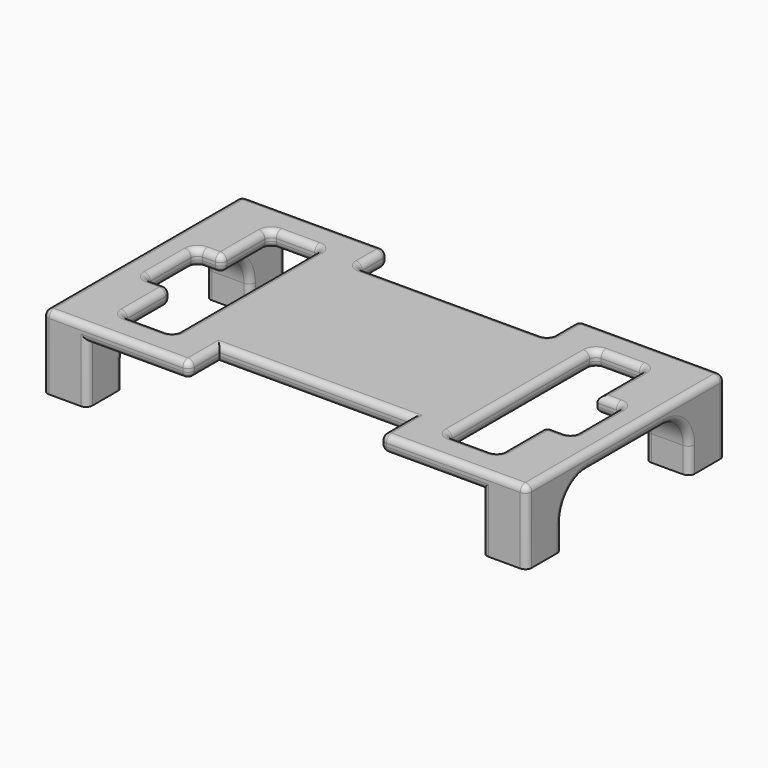
from build123d import *

# Parameters (mm, degrees)
F0_W     = 7
F0_H     = 7
F0_R     = 1.5
F0_R_2   = 1.325
F1_DEPTH = 9
F2_START = 9
F2_DEPTH = 2.5
F4_R     = 5
F5_W     = 4
F5_H     = 10
F5_W_2   = 30
F5_H_2   = 6
F6_DEPTH = 10
F7_F1_R  = 1
F7_F2_R  = 1
F7_F3_R  = 1
F7_F4_R  = 1
F7_F5_R  = 1
F7_F6_R  = 1
F7_F7_R  = 1
F7_F8_R  = 1
F7_F9_R  = 1
F7_F10_R = 1
F7_F11_R = 1
F7_F12_R = 1
F7_F13_R = 1
F7_F14_R = 1
F7_F15_R = 1
F7_F16_R = 1
F7_F17_R = 1
F7_F18_R = 1
F7_F19_R = 1
F7_F20_R = 1
F7_F21_R = 1
F7_F22_R = 1
F7_F23_R = 1
F7_F24_R = 1
F7_F25_R = 1
F7_F26_R = 1
F7_F27_R = 1
F7_F28_R = 1
F7_F29_R = 1
F7_F30_R = 1
F7_F31_R = 1
F7_F32_R = 1
F7_F33_R = 1
F7_F34_R = 1
F7_F35_R = 1
F7_F36_R = 1
F7_F37_R = 1
F7_F38_R = 1
F7_F39_R = 1
F7_F40_R = 1
F7_F41_R = 1
F7_F42_R = 1
F7_F43_R = 1
F7_F44_R = 1
F7_F45_R = 1


# Not quite as in the source:
# - a feature names something its author has since deleted; it is built from what else it names


with BuildPart() as f1:
    # F0 (on Top) → F1 (new body)
    with BuildSketch(Plane.XY):
        with Locations((-34.5, 16)):
            Rectangle(F0_W, F0_H)
        with Locations((-34.5, 16)):
            Circle(F0_R, mode=Mode.SUBTRACT)
        with Locations((-34.5, 16)):
            Circle(F0_R)
        with Locations((-34.5, 16)):
            Circle(F0_R_2, mode=Mode.SUBTRACT)
    extrude(amount=F1_DEPTH)



with BuildPart() as f1b:
    # F0 (on Top) → F1, piece 2 (new body)
    with BuildSketch(Plane.XY):
        with Locations((-34.5, -16)):
            Rectangle(F0_W, F0_H)
        with Locations((-34.5, -16)):
            Circle(F0_R_2, mode=Mode.SUBTRACT)
    extrude(amount=F1_DEPTH)


with BuildPart() as f1c:
    # F0 (on Top) → F1, piece 3 (new body)
    with BuildSketch(Plane.XY):
        with Locations((34.5, -16)):
            Rectangle(F0_W, F0_H)
        with Locations((34.5, -16)):
            Circle(F0_R_2, mode=Mode.SUBTRACT)
    extrude(amount=F1_DEPTH)


with BuildPart() as f1d:
    # F0 (on Top) → F1, piece 4 (new body)
    with BuildSketch(Plane.XY):
        with Locations((34.5, 16)):
            Rectangle(F0_W, F0_H)
        with Locations((34.5, 16)):
            Circle(F0_R_2, mode=Mode.SUBTRACT)
    extrude(amount=F1_DEPTH)


with BuildPart() as f1_1:
    add(f1.part)

    add(f1b.part)  # F2 merges F1b

    add(f1c.part)  # F2 merges F1c

    add(f1d.part)  # F2 merges F1d
    # F0 (on Top) → F2 (join)
    with BuildSketch(Plane.XY.offset(F2_START)):
        Polygon((-38, 12.5), (-38, 0), (-38, -12.5), (-31, -12.5), (-31, -19.5), (0, -19.5), (31, -19.5), (31, -12.5), (38, -12.5), (38, 0), (38, 12.5), (31, 12.5), (31, 19.5), (0, 19.5), (-31, 19.5), (-31, 12.5), align=None)
        with Locations((34.5, 16)):
            Rectangle(F0_W, F0_H)
        with Locations((34.5, 16)):
            Circle(F0_R_2, mode=Mode.SUBTRACT)
        with Locations((34.5, -16)):
            Rectangle(F0_W, F0_H)
        with Locations((34.5, -16)):
            Circle(F0_R_2, mode=Mode.SUBTRACT)
        with Locations((-34.5, 16)):
            Rectangle(F0_W, F0_H)
        with Locations((-34.5, 16)):
            Circle(F0_R, mode=Mode.SUBTRACT)
        with Locations((-34.5, 16)):
            Circle(F0_R)
        with Locations((-34.5, 16)):
            Circle(F0_R_2, mode=Mode.SUBTRACT)
        with Locations((-34.5, 16)):
            Circle(F0_R_2)
        with Locations((34.5, 16)):
            Circle(F0_R_2)
        with Locations((34.5, -16)):
            Circle(F0_R_2)
        with Locations((-34.5, -16)):
            Rectangle(F0_W, F0_H)
        with Locations((-34.5, -16)):
            Circle(F0_R_2, mode=Mode.SUBTRACT)
        with Locations((-34.5, -16)):
            Circle(F0_R_2)
    extrude(amount=F2_DEPTH)

    # F3: union 

    # F4
    f4_edges = [f1_1.edges().sort_by_distance(p)[0] for p in [
        (-34.5, -12.5, 9),
        (-34.5, 12.5, 9),
        (34.5, -12.5, 9),
        (34.5, 12.5, 9),
    ]]
    fillet(f4_edges, radius=F4_R)

    # F5 (on face) → F6 (cut)
    with BuildSketch(Plane.XY.offset(11.5)):
        Polygon((-29.5, -5), (-29.5, -14.5), (-21.5, -14.5), (-21.5, 14.5), (-29.5, 14.5), (-29.5, 5), align=None)
        with Locations((-31.5, 0)):
            Rectangle(F5_W, F5_H)
        Polygon((21.5, 14.5), (21.5, -14.5), (29.5, -14.5), (29.5, -5), (29.5, 5), (29.5, 14.5), align=None)
        with Locations((31.5, 0)):
            Rectangle(F5_W, F5_H)
        with Locations((0, -16.5)):
            Rectangle(F5_W_2, F5_H_2)
        with Locations((0, 16.5)):
            Rectangle(F5_W_2, F5_H_2)
    extrude(amount=-F6_DEPTH, mode=Mode.SUBTRACT)

    # F7: fillet of radius 1 on 100 edges, made by hand

    # F7_f1
    f7_f1_edges = [f1_1.edges().sort_by_distance(p)[0] for p in [
        (15, -19.5, 10.25),
    ]]
    fillet(f7_f1_edges, radius=F7_F1_R)

    # F7_f2
    f7_f2_edges = [f1_1.edges().sort_by_distance(p)[0] for p in [
        (-15, -19.5, 10.25),
    ]]
    fillet(f7_f2_edges, radius=F7_F2_R)

    # F7_f3
    f7_f3_edges = [f1_1.edges().sort_by_distance(p)[0] for p in [
        (-15, 19.5, 10.25),
    ]]
    fillet(f7_f3_edges, radius=F7_F3_R)

    # F7_f4
    f7_f4_edges = [f1_1.edges().sort_by_distance(p)[0] for p in [
        (-15, 13.5, 10.25),
    ]]
    fillet(f7_f4_edges, radius=F7_F4_R)

    # F7_f5
    f7_f5_edges = [f1_1.edges().sort_by_distance(p)[0] for p in [
        (15, 13.5, 10.25),
    ]]
    fillet(f7_f5_edges, radius=F7_F5_R)

    # F7_f6
    f7_f6_edges = [f1_1.edges().sort_by_distance(p)[0] for p in [
        (15, 19.5, 10.25),
    ]]
    fillet(f7_f6_edges, radius=F7_F6_R)

    # F7_f7
    f7_f7_edges = [f1_1.edges().sort_by_distance(p)[0] for p in [
        (21.5, 14.5, 10.25),
    ]]
    fillet(f7_f7_edges, radius=F7_F7_R)

    # F7_f8
    f7_f8_edges = [f1_1.edges().sort_by_distance(p)[0] for p in [
        (29.5, 14.5, 10.25),
    ]]
    fillet(f7_f8_edges, radius=F7_F8_R)

    # F7_f9
    f7_f9_edges = [f1_1.edges().sort_by_distance(p)[0] for p in [
        (33.5, 5, 10.25),
    ]]
    fillet(f7_f9_edges, radius=F7_F9_R)

    # F7_f10
    f7_f10_edges = [f1_1.edges().sort_by_distance(p)[0] for p in [
        (33.5, -5, 10.25),
    ]]
    fillet(f7_f10_edges, radius=F7_F10_R)

    # F7_f11
    f7_f11_edges = [f1_1.edges().sort_by_distance(p)[0] for p in [
        (29.5, -5, 10.25),
    ]]
    fillet(f7_f11_edges, radius=F7_F11_R)

    # F7_f12
    f7_f12_edges = [f1_1.edges().sort_by_distance(p)[0] for p in [
        (29.5, -14.5, 10.25),
    ]]
    fillet(f7_f12_edges, radius=F7_F12_R)

    # F7_f13
    f7_f13_edges = [f1_1.edges().sort_by_distance(p)[0] for p in [
        (21.5, -14.5, 10.25),
    ]]
    fillet(f7_f13_edges, radius=F7_F13_R)

    # F7_f14
    f7_f14_edges = [f1_1.edges().sort_by_distance(p)[0] for p in [
        (-29.5, -5, 10.25),
    ]]
    fillet(f7_f14_edges, radius=F7_F14_R)

    # F7_f15
    f7_f15_edges = [f1_1.edges().sort_by_distance(p)[0] for p in [
        (-33.5, -5, 10.25),
    ]]
    fillet(f7_f15_edges, radius=F7_F15_R)

    # F7_f16
    f7_f16_edges = [f1_1.edges().sort_by_distance(p)[0] for p in [
        (-33.5, 5, 10.25),
    ]]
    fillet(f7_f16_edges, radius=F7_F16_R)

    # F7_f17
    f7_f17_edges = [f1_1.edges().sort_by_distance(p)[0] for p in [
        (-29.5, 5, 10.25),
    ]]
    fillet(f7_f17_edges, radius=F7_F17_R)

    # F7_f18
    f7_f18_edges = [f1_1.edges().sort_by_distance(p)[0] for p in [
        (-29.5, 14.5, 10.25),
    ]]
    fillet(f7_f18_edges, radius=F7_F18_R)

    # F7_f19
    f7_f19_edges = [f1_1.edges().sort_by_distance(p)[0] for p in [
        (-21.5, 14.5, 10.25),
    ]]
    fillet(f7_f19_edges, radius=F7_F19_R)

    # F7_f20
    f7_f20_edges = [f1_1.edges().sort_by_distance(p)[0] for p in [
        (-21.5, -14.5, 10.25),
    ]]
    fillet(f7_f20_edges, radius=F7_F20_R)

    # F7_f21
    f7_f21_edges = [f1_1.edges().sort_by_distance(p)[0] for p in [
        (-29.5, -14.5, 10.25),
    ]]
    fillet(f7_f21_edges, radius=F7_F21_R)

    # F7_f22
    f7_f22_edges = [f1_1.edges().sort_by_distance(p)[0] for p in [
        (-31.5, 5, 11.5),
    ]]
    fillet(f7_f22_edges, radius=F7_F22_R)

    # F7_f23
    f7_f23_edges = [f1_1.edges().sort_by_distance(p)[0] for p in [
        (31.5, -5, 11.5),
    ]]
    fillet(f7_f23_edges, radius=F7_F23_R)

    # F7_f24
    f7_f24_edges = [f1_1.edges().sort_by_distance(p)[0] for p in [
        (31, 5, 9),
    ]]
    fillet(f7_f24_edges, radius=F7_F24_R)

    # F7_f25
    f7_f25_edges = [f1_1.edges().sort_by_distance(p)[0] for p in [
        (-31.5, -5, 9),
    ]]
    fillet(f7_f25_edges, radius=F7_F25_R)

    # F7_f26
    f7_f26_edges = [f1_1.edges().sort_by_distance(p)[0] for p in [
        (15, -16, 11.5),
    ]]
    fillet(f7_f26_edges, radius=F7_F26_R)

    # F7_f27
    f7_f27_edges = [f1_1.edges().sort_by_distance(p)[0] for p in [
        (15, -16, 9),
    ]]
    fillet(f7_f27_edges, radius=F7_F27_R)

    # F7_f28
    f7_f28_edges = [f1_1.edges().sort_by_distance(p)[0] for p in [
        (-15, -16, 11.5),
    ]]
    fillet(f7_f28_edges, radius=F7_F28_R)

    # F7_f29
    f7_f29_edges = [f1_1.edges().sort_by_distance(p)[0] for p in [
        (-15, -16, 9),
    ]]
    fillet(f7_f29_edges, radius=F7_F29_R)

    # F7_f30
    f7_f30_edges = [f1_1.edges().sort_by_distance(p)[0] for p in [
        (-15, 16.5, 11.5),
    ]]
    fillet(f7_f30_edges, radius=F7_F30_R)

    # F7_f31
    f7_f31_edges = [f1_1.edges().sort_by_distance(p)[0] for p in [
        (-15, 16.5, 9),
    ]]
    fillet(f7_f31_edges, radius=F7_F31_R)

    # F7_f32
    f7_f32_edges = [f1_1.edges().sort_by_distance(p)[0] for p in [
        (31, -19.5, 4.5),
    ]]
    fillet(f7_f32_edges, radius=F7_F32_R)

    # F7_f33
    f7_f33_edges = [f1_1.edges().sort_by_distance(p)[0] for p in [
        (-31, -19.5, 4.5),
    ]]
    fillet(f7_f33_edges, radius=F7_F33_R)

    # F7_f34
    f7_f34_edges = [f1_1.edges().sort_by_distance(p)[0] for p in [
        (-31, 19.5, 4.5),
    ]]
    fillet(f7_f34_edges, radius=F7_F34_R)

    # F7_f35
    f7_f35_edges = [f1_1.edges().sort_by_distance(p)[0] for p in [
        (31, 19.5, 4.5),
    ]]
    fillet(f7_f35_edges, radius=F7_F35_R)

    # F7_f36
    f7_f36_edges = [f1_1.edges().sort_by_distance(p)[0] for p in [
        (38, 19.5, 5.25),
    ]]
    fillet(f7_f36_edges, radius=F7_F36_R)

    # F7_f37
    f7_f37_edges = [f1_1.edges().sort_by_distance(p)[0] for p in [
        (-38, -19.5, 5.25),
    ]]
    fillet(f7_f37_edges, radius=F7_F37_R)

    # F7_f38
    f7_f38_edges = [f1_1.edges().sort_by_distance(p)[0] for p in [
        (31, 12.5, 2),
        (31, 11.0355339059, 7.5355339059),
    ]]
    fillet(f7_f38_edges, radius=F7_F38_R)

    # F7_f39
    f7_f39_edges = [f1_1.edges().sort_by_distance(p)[0] for p in [
        (-31, 12.5, 2),
        (-31, 11.0355339059, 7.5355339059),
    ]]
    fillet(f7_f39_edges, radius=F7_F39_R)

    # F7_f40
    f7_f40_edges = [f1_1.edges().sort_by_distance(p)[0] for p in [
        (31, -12.5, 2),
        (31, -11.0355339059, 7.5355339059),
    ]]
    fillet(f7_f40_edges, radius=F7_F40_R)

    # F7_f41
    f7_f41_edges = [f1_1.edges().sort_by_distance(p)[0] for p in [
        (-31, -12.5, 2),
        (-31, -11.0355339059, 7.5355339059),
    ]]
    fillet(f7_f41_edges, radius=F7_F41_R)

    # F7_f42
    f7_f42_edges = [f1_1.edges().sort_by_distance(p)[0] for p in [
        (0, -13.5, 11.5),
    ]]
    fillet(f7_f42_edges, radius=F7_F42_R)

    # F7_f43
    f7_f43_edges = [f1_1.edges().sort_by_distance(p)[0] for p in [
        (0, -13.5, 9),
    ]]
    fillet(f7_f43_edges, radius=F7_F43_R)

    # F7_f44
    f7_f44_edges = [f1_1.edges().sort_by_distance(p)[0] for p in [
        (38, 12.5, 2),
        (38, 11.0355339059, 7.5355339059),
        (38, 0, 9),
        (38, -11.0355339059, 7.5355339059),
        (38, -12.5, 2),
    ]]
    fillet(f7_f44_edges, radius=F7_F44_R)

    # F7_f45
    f7_f45_edges = [f1_1.edges().sort_by_distance(p)[0] for p in [
        (-38, -11.0355339059, 7.5355339059),
        (-38, -12.5, 2),
        (-38, 0, 9),
        (-38, 11.0355339059, 7.5355339059),
        (-38, 12.5, 2),
    ]]
    fillet(f7_f45_edges, radius=F7_F45_R)


solid = f1_1.part
